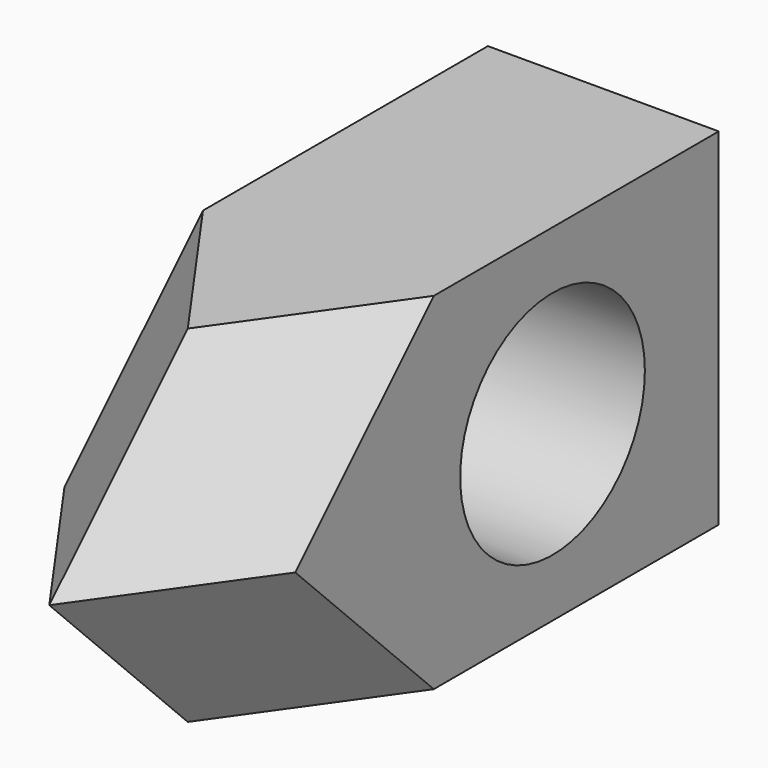
from build123d import *

# Parameters (mm, degrees)
F0_W      = 12.7
F0_H      = 19.05
F1_DEPTH  = 12.7
F2_W      = 12.7
F2_H      = 19.05
F3_DEPTH  = 12.7
F4_SIZE   = 9.52499
F5_SIZE   = 6.35
F5_SIZE_2 = 6.34999
F6_R      = 6.35
F7_DEPTH  = 12.7


# Not quite as in the source:
# - a fillet or chamfer is up to 0.001 mm smaller than in the source, because OpenCascade refuses the exact size


with BuildPart() as f1:
    # F0 (on Front) → F1 (new body, symmetric)
    with BuildSketch(Plane.XZ):
        Rectangle(F0_W, F0_H)
    extrude(amount=F1_DEPTH, both=True)

    # F2 (on face) → F3 (join)
    with BuildSketch(Plane.XZ.offset(12.7)):
        Rectangle(F2_W, F2_H)
    extrude(amount=F3_DEPTH)

    # F4 (size 9.525 in the source; OpenCascade refuses exactly that, so slightly less here)
    f4_edges = [f1.edges().sort_by_distance(p)[0] for p in [
        (0, -25.4, 9.525),
        (0, -25.4, -9.525),
    ]]
    chamfer(f4_edges, length=F4_SIZE)

    # F5 (call 1 of 4: OpenCascade refuses the feature's edges together)
    f5_edges = [f1.edges().sort_by_distance(p)[0] for p in [
        (-6.35, -20.637505, 4.762505),
    ]]
    chamfer(f5_edges, length=F5_SIZE)

    # F5#2 (call 2 of 4)
    f5_2_edges = [f1.edges().sort_by_distance(p)[0] for p in [
        (-6.35, -20.637505, -4.762505),
    ]]
    chamfer(f5_2_edges, length=F5_SIZE)

    # F5#3 (call 3 of 4) (size 6.35 in the source; OpenCascade refuses exactly that, so slightly less here)
    f5_3_edges = [f1.edges().sort_by_distance(p)[0] for p in [
        (6.35, -20.637505, 4.762505),
    ]]
    chamfer(f5_3_edges, length=F5_SIZE_2)

    # F5#4 (call 4 of 4) (size 6.35 in the source; OpenCascade refuses exactly that, so slightly less here)
    f5_4_edges = [f1.edges().sort_by_distance(p)[0] for p in [
        (6.35, -20.637505, -4.762505),
    ]]
    chamfer(f5_4_edges, length=F5_SIZE_2)

    # F6 (on face) → F7 (cut)
    with BuildSketch(Plane.YZ.offset(6.35)):
        with Locations((1.27, 0)):
            Circle(F6_R)
    extrude(amount=-F7_DEPTH, mode=Mode.SUBTRACT)


solid = f1.part
